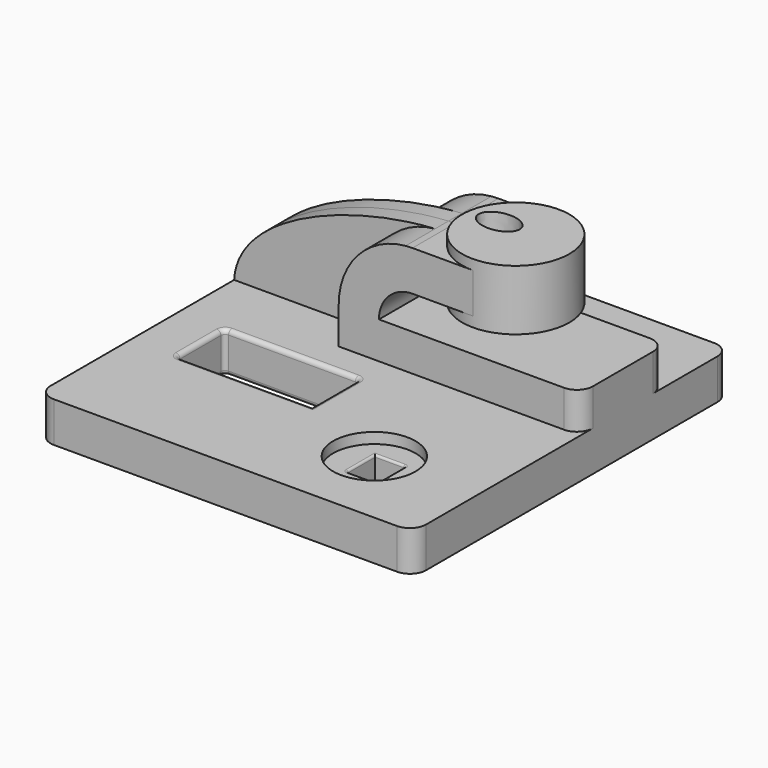
from build123d import *

# Parameters (mm, degrees)
F1_DEPTH  = 63.5
F0_W      = 25.4
F0_H      = 19.05
F2_DEPTH  = 25.4
F3_DEPTH  = 7.9375
F5_DEPTH  = 95.25
F6_DEPTH  = 60.706
F7_W      = 64.0991125256
F7_H      = 28.2470658422
F8_DEPTH  = 25.4
F9_R      = 19.5079134093
F10_DEPTH = 5.08
F11_W     = 14.4394114614
F11_H     = 16.9663056731
F12_DEPTH = 25.4
F14_DEPTH = 28.575
F15_R     = 7.62
F16_R     = 2.032
F17_R     = 1.016


with BuildPart() as f1:
    # F0 (on Front) → F1 (new body, symmetric)
    with BuildSketch(Plane.XZ):
        Polygon((22.225, 9.525), (-41.275, 9.525), (-41.275, -9.525), (41.275, -9.525), (41.275, 9.525), align=None)
    extrude(amount=F1_DEPTH, both=True)

    # F0 (on Front) → F2 (join, symmetric)
    with BuildSketch(Plane.XZ):
        with BuildLine():
            Line((22.225, 27.0002), (22.225, 9.525))
            Line((22.225, 9.525), (41.275, 9.525))
            Line((41.275, 9.525), (41.275, 27.0002))
            ThreePointArc((41.275, 27.0002), (45.9246798487, 38.2255201513), (57.15, 42.8752))
            Line((57.15, 42.8752), (60.325, 42.8752))
            Line((60.325, 42.8752), (60.325, 61.9252))
            Line((60.325, 61.9252), (57.15, 61.9252))
            add(Edge.make_bspline(
                [(53.8854342407, 61.7722898912), (54.9842067368, 61.8365871986), (56.0728453275, 61.8876096574), (57.15, 61.9252)],
                knots=[108.5245810491, 108.5245810491, 108.5245810491, 108.5245810491, 111.5045361635, 111.5045361635, 111.5045361635, 111.5045361635], degree=3))
            ThreePointArc((53.8854342407, 61.7722898912), (31.3258777096, 50.5133948686), (22.225, 27.0002))
        make_face()
        with Locations((73.025, 52.4002)):
            Rectangle(F0_W, F0_H)
    extrude(amount=F2_DEPTH, both=True)

    # F0 (on Front) → F3 (join, symmetric)
    with BuildSketch(Plane.XZ):
        with BuildLine():
            add(Edge.make_bspline(
                [(-41.275, 9.525), (-39.5856284224, 39.4828766469), (13.870125209, 59.4306981306), (53.8854342407, 61.7722898912)],
                knots=[0, 0, 0, 0, 108.5245810491, 108.5245810491, 108.5245810491, 108.5245810491], degree=3))
            Line((-41.275, 9.525), (22.225, 9.525))
            Line((22.225, 9.525), (22.225, 27.0002))
            ThreePointArc((22.225, 27.0002), (31.3258777096, 50.5133948686), (53.8854342407, 61.7722898912))
        make_face()
    extrude(amount=F3_DEPTH, both=True)

    # F0 (on Front) → F4 (revolve)
    with BuildSketch(Plane.XZ):
        Polygon((85.725, 66.675), (85.725, 61.9252), (85.725, 42.8752), (85.725, 38.1), (111.125, 38.1), (111.125, 66.675), align=None)
    revolve(axis=Axis((85.725, 0, 52.3875), (0, 0, 1)))

    # F5 (add): a face of the model
    f5_faces = [f1.faces().sort_by_distance(p)[0] for p in [
        (41.275, 0, 4.9023288334),
    ]]
    extrude(f5_faces, amount=F5_DEPTH)

    # F6 (add): a face of the model
    f6_faces = [f1.faces().sort_by_distance(p)[0] for p in [
        (47.625, -63.5, 0),
    ]]
    extrude(f6_faces, amount=F6_DEPTH)

    # F7 (on face) → F8 (cut)
    with BuildSketch(Plane.XY.offset(9.525)):
        with Locations((12.3161775991, -54.8000894487)):
            Rectangle(F7_W, F7_H)
    extrude(amount=-F8_DEPTH, mode=Mode.SUBTRACT)

    # F9 (on face) → F10 (cut)
    with BuildSketch(Plane.XY.offset(9.525)):
        with Locations((87.4239131329, -85.8199995224)):
            Circle(F9_R)
    extrude(amount=-F10_DEPTH, mode=Mode.SUBTRACT)

    # F11 (on face) → F12 (cut)
    with BuildSketch(Plane.XY.offset(9.525)):
        with Locations((88.0553610623, -85.5649597943)):
            Rectangle(F11_W, F11_H)
    extrude(amount=-F12_DEPTH, mode=Mode.SUBTRACT)

    # F13 (on face) → F14 (cut, through all)
    with BuildSketch(Plane.XY.offset(66.675)):
        with BuildLine():
            add(Edge.make_bspline(
                [(84.4615474343, 3.9708414115), (84.4615474343, 15.3508284031), (69.8416419327, 9.6608349073), (55.2217364311, 3.9708414115), (69.8416419327, -1.7191520843), (84.4615474343, -7.4091455801), (84.4615474343, 3.9708414115)],
                knots=[0, 0, 0, 2.0943951024, 2.0943951024, 4.1887902048, 4.1887902048, 6.2831853072, 6.2831853072, 6.2831853072], degree=2, weights=[1, 0.5, 1, 0.5, 1, 0.5, 1]))
        make_face()
    extrude(amount=-F14_DEPTH, mode=Mode.SUBTRACT)

    # F15
    f15_edges = [f1.edges().sort_by_distance(p)[0] for p in [
        (-41.275, -124.206, 0),
        (136.525, -124.206, 0),
        (136.525, -25.4, 18.2626),
        (136.525, 25.4, 18.2626),
        (136.525, 63.5, 0),
    ]]
    fillet(f15_edges, radius=F15_R)

    # F16
    f16_edges = [f1.edges().sort_by_distance(p)[0] for p in [
        (-19.733379, -54.800089, 9.525),
        (-19.733379, -68.923622, 0),
        (-19.733379, -54.800089, -9.525),
        (-19.733379, -40.676557, 0),
        (12.316178, -40.676557, 9.525),
        (12.316178, -40.676557, -9.525),
        (44.365734, -40.676557, 0),
        (12.316178, -68.923622, -9.525),
        (44.365734, -54.800089, -9.525),
        (12.316178, -68.923622, 9.525),
        (44.365734, -54.800089, 9.525),
    ]]
    fillet(f16_edges, radius=F16_R)

    # F17
    f17_edges = [f1.edges().sort_by_distance(p)[0] for p in [
        (88.055361, -77.081807, 4.445),
        (95.275067, -85.56496, 4.445),
        (95.275067, -77.081807, -2.54),
        (95.275067, -85.56496, -9.525),
        (95.275067, -94.048113, -2.54),
        (80.835655, -85.56496, 4.445),
        (88.055361, -94.048113, 4.445),
        (88.055361, -94.048113, -9.525),
        (80.835655, -94.048113, -2.54),
        (80.835655, -85.56496, -9.525),
        (88.055361, -77.081807, -9.525),
    ]]
    fillet(f17_edges, radius=F17_R)


solid = f1.part
